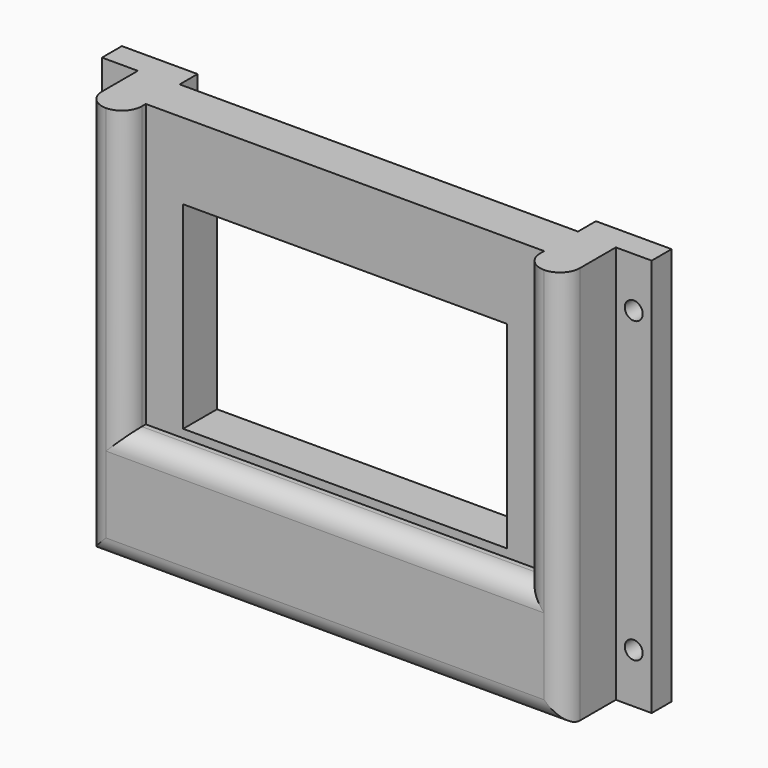
from build123d import *

# Parameters (mm, degrees)
F0_W     = 101.6
F0_H     = 101.6
F0_W_2   = 82.55
F0_H_2   = 50.419
F1_DEPTH = 10.795
F2_W     = 101.6
F2_H     = 29.6545
F2_W_2   = 82.55
F2_H_2   = 19.05
F3_DEPTH = 6.35
F4_W     = 10.16
F4_H     = 101.6
F5_DEPTH = 22.86
F6_W     = 9.144
F6_H     = 101.6
F6_R     = 2.286
F7_DEPTH = 6.35
F8_R     = 5.08
F9_R     = 5.07999


# Not quite as in the source:
# - a fillet or chamfer is up to 0.001 mm smaller than in the source, because OpenCascade refuses the exact size


with BuildPart() as f1:
    # F0 (on Front) → F1 (new body)
    with BuildSketch(Plane.XZ):
        with Locations((0, -6.1595)):
            Rectangle(F0_W, F0_H)
        Polygon((-41.275, -29.0195), (0, -29.0195), (41.275, -29.0195), (41.275, -48.0695), (-41.275, -48.0695), align=None, mode=Mode.SUBTRACT)
        Rectangle(F0_W_2, F0_H_2, mode=Mode.SUBTRACT)
    extrude(amount=F1_DEPTH)

    # F2 (on face) → F3 (join)
    with BuildSketch(Plane.XZ.offset(10.795)):
        with Locations((0, -42.13225)):
            Rectangle(F2_W, F2_H)
        with Locations((0, -38.5445)):
            Rectangle(F2_W_2, F2_H_2, mode=Mode.SUBTRACT)
        with Locations((0, -38.5445)):
            Rectangle(F2_W_2, F2_H_2)
    extrude(amount=F3_DEPTH)

    # F4 (on face) → F5 (join)
    with BuildSketch(Plane.XZ.offset(17.145)):
        with Locations((-55.88, -6.1595)):
            Rectangle(F4_W, F4_H)
        with Locations((55.88, -6.1595)):
            Rectangle(F4_W, F4_H)
    extrude(amount=-F5_DEPTH)

    # F6 (on face) → F7 (join)
    with BuildSketch(Plane(origin=(0, 5.715, 0), x_dir=(-1, 0, 0), z_dir=(0, 1, 0))):
        with Locations((-65.532, -6.1595)):
            Rectangle(F6_W, F6_H)
        with Locations((-65.532, -44.2595)):
            Circle(F6_R, mode=Mode.SUBTRACT)
        with Locations((-65.532, 31.9405)):
            Circle(F6_R, mode=Mode.SUBTRACT)
        with Locations((65.532, -6.1595)):
            Rectangle(F6_W, F6_H)
        with Locations((65.532, -44.2595)):
            Circle(F6_R, mode=Mode.SUBTRACT)
        with Locations((65.532, 31.9405)):
            Circle(F6_R, mode=Mode.SUBTRACT)
    extrude(amount=-F7_DEPTH)

    # F8
    f8_edges = [f1.edges().sort_by_distance(p)[0] for p in [
        (-60.96, -17.145, -6.1595),
        (0, -17.145, -56.9595),
        (60.96, -17.145, -6.1595),
    ]]
    fillet(f8_edges, radius=F8_R)

    # F9 (radius 5.08 in the source; OpenCascade refuses exactly that, so slightly less here)
    f9_edges = [f1.edges().sort_by_distance(p)[0] for p in [
        (-50.8, -17.145, 8.66775),
        (0, -17.145, -27.305),
        (50.8, -17.145, 8.66775),
    ]]
    fillet(f9_edges, radius=F9_R)


solid = f1.part
